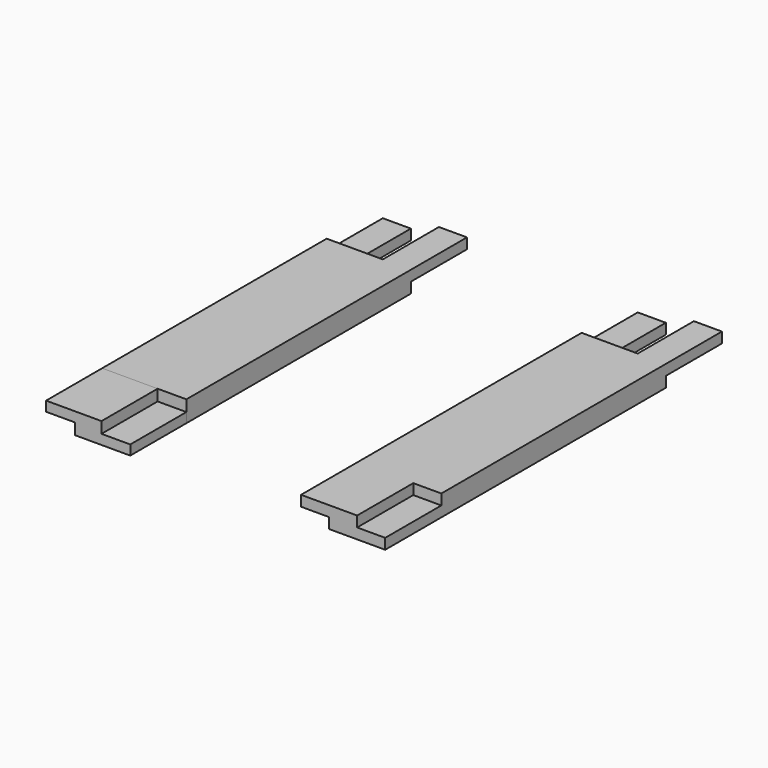
from build123d import *

# Parameters (mm, degrees)
F0_W     = 12
F0_H     = 40
F1_DEPTH = 3
F4_DEPTH = 10
F6_W     = 4
F6_H     = 1.5
F7_DEPTH = 10
F5_W     = 4
F5_H     = 1.5


# Not quite as in the source:
# - a feature names something its author has since deleted; it is built from what else it names


with BuildPart() as f1:
    # F0 (on Top) → F1 (new body)
    with BuildSketch(Plane.XY):
        with Locations((-22.7465788424, 20)):
            Rectangle(F0_W, F0_H)
    extrude(amount=F1_DEPTH)

    # F6 (on face) → F7 (join)
    with BuildSketch(Plane(origin=(0, 40, 0), x_dir=(-1, 0, 0), z_dir=(0, 1, 0))):
        with Locations((18.7465788424, 2.25)):
            Rectangle(F6_W, F6_H)
        with Locations((26.7465788424, 0.75)):
            Rectangle(F6_W, F6_H)
    extrude(amount=F7_DEPTH)


with BuildPart() as f1b:
    # F0 (on Top) → F1, piece 2 (new body)
    with BuildSketch(Plane.XY):
        with Locations((13.5962403789, 20)):
            Rectangle(F0_W, F0_H)
    extrude(amount=F1_DEPTH)

    # F3 (on face) → F4 (join)
    with BuildSketch(Plane.XZ):
        Polygon((15.5962403789, 3), (7.5962403789, 3), (7.5962403789, 1.5), (11.5962403789, 1.5), (11.5962403789, 0), (19.5962403789, 0), (19.5962403789, 1.5), (15.5962403789, 1.5), align=None)
    extrude(amount=F4_DEPTH)

    # F5 (on face) → F7, piece 2 (join)
    with BuildSketch(Plane(origin=(0, 40, 0), x_dir=(-1, 0, 0), z_dir=(0, 1, 0))):
        with Locations((-17.5962403789, 2.25)):
            Rectangle(F5_W, F5_H)
        with Locations((-9.5962403789, 0.75)):
            Rectangle(F5_W, F5_H)
    extrude(amount=F7_DEPTH)


with BuildPart() as f4:
    # F2 (on face) → F4, piece 2 (new body)
    with BuildSketch(Plane.XZ):
        Polygon((-20.8465788424, 3), (-28.7465788424, 3), (-28.7465788424, 1.6), (-24.6465788424, 1.6), (-24.6465788424, 0), (-16.7465788424, 0), (-16.7465788424, 1.4), (-20.8465788424, 1.4), align=None)
    extrude(amount=F4_DEPTH)


solid = Compound([f1.part, f1b.part, f4.part])
